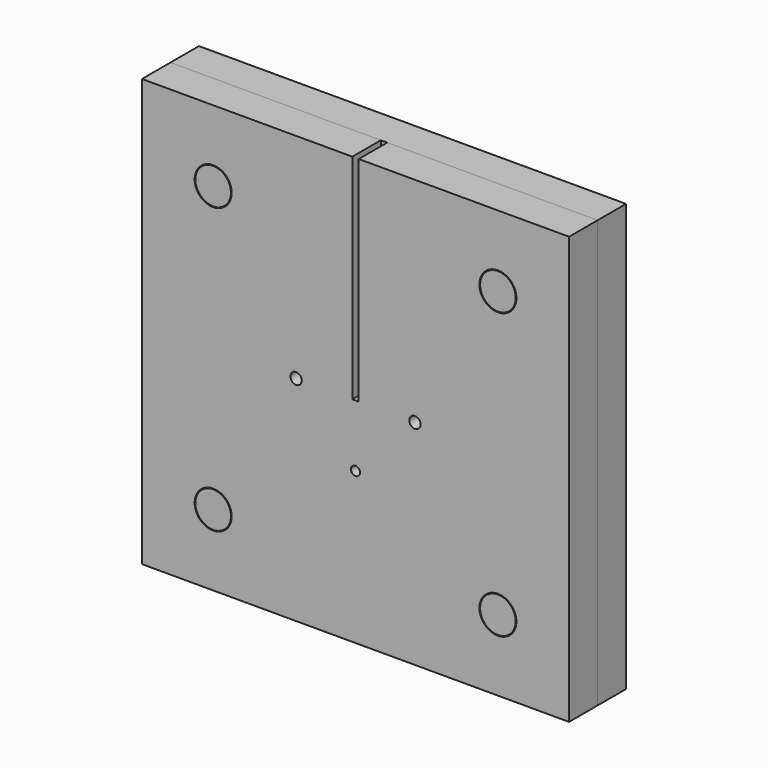
from build123d import *

# Parameters (mm, degrees)
F0_W      = 60
F0_H      = 60
F1_DEPTH  = 2.5
F2_R      = 8.15
F3_DEPTH  = 1.2
F4_R      = 7.1
F5_DEPTH  = 2.5
F6_R      = 2.5
F7_DEPTH  = 5
F8_W      = 60
F8_H      = 60
F8_R      = 2.6
F9_DEPTH  = 5
F10_R     = 9.675
F11_DEPTH = 1.1
F12_W     = 0.9
F12_H     = 32.9937078059
F13_DEPTH = 25
F14_R     = 0.8
F15_DEPTH = 25
F16_R     = 0.6352054313
F17_DEPTH = 25


with BuildPart() as f1:
    # F0 (on Front) → F1 (new body, symmetric)
    with BuildSketch(Plane.XZ):
        Rectangle(F0_W, F0_H)
    extrude(amount=F1_DEPTH, both=True)

    # F2 (on face) → F3 (cut)
    with BuildSketch(Plane.XZ.offset(2.5)):
        Circle(F2_R)
    extrude(amount=-F3_DEPTH, mode=Mode.SUBTRACT)

    # F4 (on face) → F5 (join)
    with BuildSketch(Plane.XZ.offset(1.3)):
        Circle(F4_R)
    extrude(amount=F5_DEPTH)

    # F6 (on face) → F7 (join)
    with BuildSketch(Plane.XZ.offset(2.5)):
        with Locations((-20, 20)):
            Circle(F6_R)
        with Locations((20, 20)):
            Circle(F6_R)
        with Locations((20, -20)):
            Circle(F6_R)
        with Locations((-20, -20)):
            Circle(F6_R)
    extrude(amount=F7_DEPTH)


with BuildPart() as f9:
    # F8 (on face) → F9 (new body)
    with BuildSketch(Plane.XZ.offset(2.5)):
        Rectangle(F8_W, F8_H)
        with Locations((-20, -20)):
            Circle(F8_R, mode=Mode.SUBTRACT)
        with Locations((20, -20)):
            Circle(F8_R, mode=Mode.SUBTRACT)
        with Locations((-20, 20)):
            Circle(F8_R, mode=Mode.SUBTRACT)
        with Locations((20, 20)):
            Circle(F8_R, mode=Mode.SUBTRACT)
    extrude(amount=F9_DEPTH)

    # F10 (on face) → F11 (cut)
    with BuildSketch(Plane(origin=(0, -2.5, 0), x_dir=(-1, 0, 0), z_dir=(0, 1, 0))):
        Circle(F10_R)
    extrude(amount=-F11_DEPTH, mode=Mode.SUBTRACT)

    # F12 (on face) → F13 (cut)
    with BuildSketch(Plane.XZ.offset(7.5)):
        with Locations((0, 16.4968539029)):
            Rectangle(F12_W, F12_H)
    extrude(amount=-F13_DEPTH, mode=Mode.SUBTRACT)

    # F14 (on face) → F15 (cut)
    with BuildSketch(Plane.XZ.offset(7.5)):
        with Locations((-8.35, 0)):
            Circle(F14_R)
        with Locations((8.35, 0)):
            Circle(F14_R)
    extrude(amount=-F15_DEPTH, mode=Mode.SUBTRACT)

    # F16 (on face) → F17 (cut)
    with BuildSketch(Plane.XZ.offset(7.5)):
        with Locations((0, -8.7182717398)):
            Circle(F16_R)
    extrude(amount=-F17_DEPTH, mode=Mode.SUBTRACT)


solid = Compound([f1.part, f9.part])
